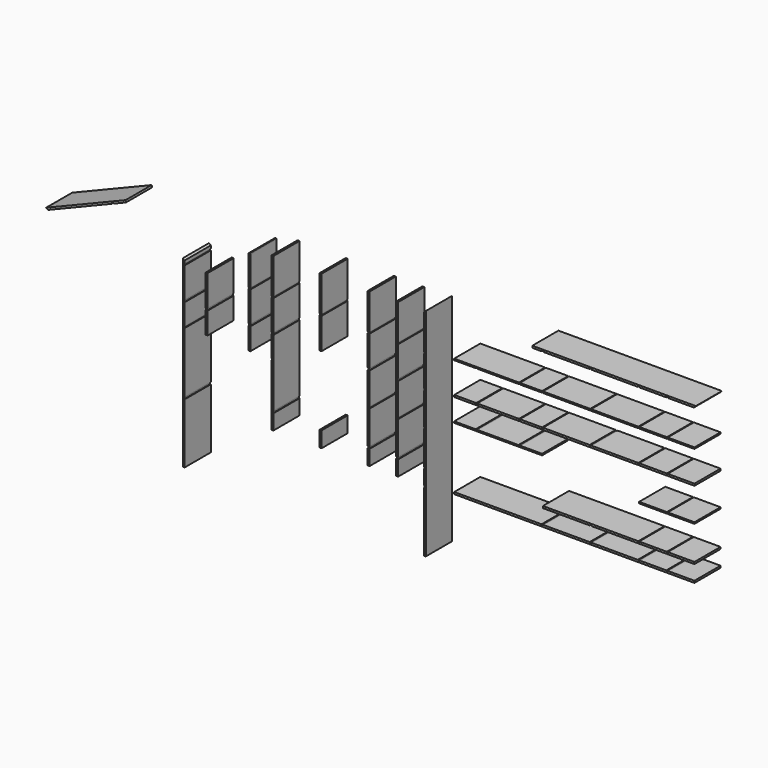
from build123d import *

# Parameters (mm, degrees)
F1_DEPTH = 400
F4_DEPTH = 400
F5_DEPTH = 400


# Not quite as in the source:
# - a feature names something its author has since deleted; it is built from what else it names


with BuildPart() as f1:
    # F0 (on Front) → F1 (new body)
    with BuildSketch(Plane.XZ):
        Polygon((0, 2251), (0, 0), (24, 0), (24, 502), (24, 735), (17, 735), (17, 759), (24, 759), (24, 1504.2), (17, 1504.2), (17, 1522.2), (24, 1522.2), (24, 1783), (17, 1783), (17, 1807), (24, 1807), (24, 2181), (17, 2181), (17, 2199), (24, 2199), (24, 2234.8896542695), align=None)
    extrude(amount=F1_DEPTH)


with BuildPart() as f1b:
    # F0 (on Front) → F1, piece 2 (new body)
    with BuildSketch(Plane.XZ):
        Polygon((2980, 0), (2980, 2650), (2956, 2626), (2956, 2249), (2956, 2199), (2963, 2199), (2963, 2181), (2956, 2181), (2956, 1807), (2963, 1807), (2963, 1783), (2956, 1783), (2956, 1390.5), (2963, 1390.5), (2963, 1372.5), (2956, 1372.5), (2956, 962), (2963, 962), (2963, 938), (2956, 938), (2956, 759), (2963, 759), (2963, 735), (2956, 735), (2956, 550), (2956, 526), (2956, 502), (2956, 0), align=None)
    extrude(amount=F1_DEPTH)


with BuildPart() as f1c:
    # F0 (on Front) → F1, piece 3 (new body)
    with BuildSketch(Plane.XZ):
        Polygon((804.639455329, 2565.1562908123), (804.639455329, 2554.3513390656), (804.6394553291, 2249), (804.6394553291, 2199), (811.639455329, 2199), (811.639455329, 2181), (804.6394553291, 2181), (804.6394553293, 1807), (811.639455329, 1807), (811.639455329, 1783), (804.6394553293, 1783), (804.6394553294, 1522.2), (804.6394553294, 1515.2), (828.6394553284, 1515.2), (828.6394553284, 1522.2), (828.6394553285, 1783), (821.6394553285, 1783), (821.6394553285, 1807), (828.6394553285, 1807), (828.6394553288, 2181), (821.6394553288, 2181), (821.6394553288, 2199), (828.6394553288, 2199), (828.6394553288, 2249), (828.639455329, 2564.1728775272), (824.8520180611, 2573.4278934073), align=None)
    extrude(amount=F1_DEPTH)


with BuildPart() as f1d:
    # F0 (on Front) → F1, piece 4 (new body)
    with BuildSketch(Plane.XZ):
        Polygon((1088, 2636), (1088, 2626), (1088, 2249), (1088, 2199), (1095, 2199), (1095, 2181), (1088, 2181), (1088, 1807), (1095, 1807), (1095, 1783), (1088, 1783), (1088, 1522.1999999999), (1095, 1522.1999999998), (1095, 1504.2), (1088, 1504.2), (1088, 1222.6), (1088, 938), (1088, 759), (1088, 752), (1112, 752), (1112, 759), (1112, 938), (1105, 938), (1105, 962), (1112, 962), (1112, 1222.6), (1112, 1783), (1105, 1783), (1105, 1807), (1112, 1807), (1112, 2181), (1105, 2181), (1105, 2199), (1112, 2199), (1112, 2249), (1112, 2626), (1112, 2636), align=None)
    extrude(amount=F1_DEPTH)


with BuildPart() as f1e:
    # F0 (on Front) → F1, piece 5 (new body)
    with BuildSketch(Plane.XZ):
        Polygon((2642, 2249), (2642, 2626), (2642, 2636), (2618, 2636), (2618, 2626), (2618, 2249), (2618, 2199), (2625, 2199), (2625, 2181), (2618, 2181), (2618, 1807), (2625, 1807), (2625, 1783), (2618, 1783), (2618, 1390.5), (2625, 1390.5), (2625, 1372.5), (2618, 1372.5), (2618, 962), (2625, 962), (2625, 938), (2618, 938), (2618, 759), (2618, 752), (2642, 752), (2642, 759), (2642, 938), (2635, 938), (2635, 962), (2642, 962), (2642, 1372.5), (2635, 1372.5), (2635, 1390.5), (2642, 1390.5), (2642, 1783), (2635, 1783), (2635, 1807), (2642, 1807), (2642, 2181), (2635, 2181), (2635, 2199), (2642, 2199), align=None)
    extrude(amount=F1_DEPTH)


with BuildPart() as f1f:
    # F0 (on Front) → F1, piece 6 (new body)
    with BuildSketch(Plane.XZ):
        Polygon((280.5054049087, 2188), (280.5054049087, 2181), (280.5054049087, 1807), (287.5054049087, 1807), (287.5054049087, 1783), (280.5054049087, 1783), (280.5054049087, 1522.2), (280.5054049087, 1515.2), (304.5054049087, 1515.2), (304.5054049087, 1522.2), (304.5054049087, 1783), (297.5054049087, 1783), (297.5054049087, 1807), (304.5054049087, 1807), (304.5054049087, 2181), (304.5054049087, 2188), align=None)
    extrude(amount=F1_DEPTH)


with BuildPart() as f1g:
    # F0 (on Front) → F1, piece 7 (new body)
    with BuildSketch(Plane.XZ):
        Polygon((1678, 2636), (1678, 2626), (1678, 2249), (1678, 2199), (1685, 2199), (1685, 2181), (1678, 2181), (1678, 1807), (1678, 1800), (1702, 1800), (1702, 1807), (1702, 2181), (1695, 2181), (1695, 2199), (1702, 2199), (1702, 2249), (1702, 2626), (1702, 2636), align=None)
    extrude(amount=F1_DEPTH)


with BuildPart() as f1h:
    # F0 (on Front) → F1, piece 8 (new body)
    with BuildSketch(Plane.XZ):
        Polygon((2291.9720954895, 2249), (2291.9720954895, 2626), (2291.9720954895, 2636), (2268, 2636), (2268, 2626), (2268, 2249), (2268, 2199), (2275, 2199), (2275, 2181), (2268, 2181), (2268, 1807), (2275, 1807), (2275, 1783), (2268, 1783), (2268, 962), (2275, 962), (2275, 938), (2268, 938), (2268, 759), (2268, 752), (2292, 752), (2292, 759), (2292, 938), (2284.9720954895, 938), (2284.9720954895, 962), (2292, 962), (2292, 1372.5), (2284.9720954895, 1372.5), (2284.9720954895, 1390.5), (2292, 1390.5), (2292, 1783), (2284.9720954895, 1783), (2284.9720954895, 1807), (2291.9720954895, 1807), (2291.9720954895, 2181), (2284.9720954895, 2181), (2284.9720954895, 2199), (2291.9720954895, 2199), align=None)
    extrude(amount=F1_DEPTH)


with BuildPart() as f1i:
    # F0 (on Front) → F1, piece 9 (new body)
    with BuildSketch(Plane.XZ):
        Polygon((1678, 938), (1678, 759), (1678, 752), (1702, 752), (1702, 759), (1702, 938), (1702, 945), (1678, 945), align=None)
    extrude(amount=F1_DEPTH)


with BuildPart() as f4:
    # F3 (on Front) → F4 (new body)
    with BuildSketch(Plane.XZ):
        Polygon((-701.0374307632, 2650), (-1676.0374307632, 2251), (-1652.0374307632, 2234.8896542695), (-871.3979754343, 2554.3513390656), (-871.3979754343, 2565.1562908123), (-851.1854127022, 2573.4278934073), (-847.3979754343, 2564.1728775272), (-696.3166611209, 2626), align=None)
    extrude(amount=F4_DEPTH)


with BuildPart() as f5:
    # F2 (on Front) → F5 (new body)
    with BuildSketch(Plane.XZ):
        Polygon((6291.6567134857, 2700.713174873), (4286.6567134857, 2700.713174873), (4289.0170983069, 2688.713174873), (4291.377483128, 2676.713174873), (4399.6567134857, 2676.713174873), (4399.6567134857, 2686.713174873), (4423.6567134857, 2686.713174873), (4423.6567134857, 2676.713174873), (4989.6567134857, 2676.713174873), (4989.6567134857, 2686.713174873), (5013.6567134857, 2686.713174873), (5013.6567134857, 2676.713174873), (5579.6567134857, 2676.713174873), (5579.6567134857, 2686.713174873), (5603.6288089752, 2686.713174873), (5603.6288089752, 2676.713174873), (5929.6567134857, 2676.713174873), (5929.6567134857, 2686.713174873), (5953.6567134857, 2686.713174873), (5953.6567134857, 2676.713174873), (6267.6567134857, 2676.713174873), align=None)
    extrude(amount=F5_DEPTH)


with BuildPart() as f5b:
    # F2 (on Front) → F5, piece 2 (new body)
    with BuildSketch(Plane.XZ):
        Polygon((5953.6567134857, 988.713174873), (6267.6567134857, 988.713174873), (6274.6567134857, 988.713174873), (6274.6567134857, 1012.713174873), (6267.6567134857, 1012.713174873), (6129.7695007324, 1012.713174873), (5953.6567134857, 1012.713174873), (5946.6567134857, 1012.713174873), (5946.6567134857, 988.713174873), align=None)
    extrude(amount=F5_DEPTH)


with BuildPart() as f5c:
    # F2 (on Front) → F5, piece 3 (new body)
    with BuildSketch(Plane.XZ):
        Polygon((5603.6567134857, 988.713174873), (5929.6567134857, 988.713174873), (5936.6567134857, 988.713174873), (5936.6567134857, 1012.713174873), (5929.6567134857, 1012.713174873), (5603.6567134857, 1012.713174873), (5596.6288089752, 1012.713174873), (5596.6288089752, 988.713174873), align=None)
    extrude(amount=F5_DEPTH)


with BuildPart() as f5d:
    # F2 (on Front) → F5, piece 4 (new body)
    with BuildSketch(Plane.XZ):
        Polygon((4416.6567134857, 988.713174873), (4423.6567134857, 988.713174873), (4989.6567134857, 988.713174873), (4989.6567134857, 995.713174873), (5013.6567134857, 995.713174873), (5013.6567134857, 988.713174873), (5579.6567134857, 988.713174873), (5586.6567134857, 988.713174873), (5586.6567134857, 1012.713174873), (5579.6567134857, 1012.713174873), (4423.6567134857, 1012.713174873), (4416.6567134857, 1012.713174873), align=None)
    extrude(amount=F5_DEPTH)


with BuildPart() as f5e:
    # F2 (on Front) → F5, piece 5 (new body)
    with BuildSketch(Plane.XZ):
        Polygon((5603.6567134857, 1423.213174873), (5929.6567134857, 1423.213174873), (5936.6567134857, 1423.213174873), (5936.6567134857, 1441.213174873), (5929.6567134857, 1441.213174873), (5603.6567134857, 1441.213174873), (5596.6288089752, 1441.213174873), (5596.6288089752, 1423.213174873), align=None)
    extrude(amount=F5_DEPTH)


with BuildPart() as f5f:
    # F2 (on Front) → F5, piece 6 (new body)
    with BuildSketch(Plane.XZ):
        Polygon((5953.6567134857, 1423.213174873), (6267.6567134857, 1423.213174873), (6274.6567134857, 1423.213174873), (6274.6567134857, 1441.213174873), (6267.6567134857, 1441.213174873), (5953.6567134857, 1441.213174873), (5946.6567134857, 1441.213174873), (5946.6567134857, 1423.213174873), align=None)
    extrude(amount=F5_DEPTH)


with BuildPart() as f5g:
    # F2 (on Front) → F5, piece 7 (new body)
    with BuildSketch(Plane.XZ):
        Polygon((6274.6567134857, 1857.713174873), (6267.6567134857, 1857.713174873), (5953.6567134857, 1857.713174873), (5946.6567134857, 1857.713174873), (5946.6567134857, 1833.713174873), (5953.6567134857, 1833.713174873), (6129.7695007324, 1833.713174873), (6267.6567134857, 1833.713174873), (6274.6567134857, 1833.713174873), align=None)
    extrude(amount=F5_DEPTH)


with BuildPart() as f5h:
    # F2 (on Front) → F5, piece 8 (new body)
    with BuildSketch(Plane.XZ):
        Polygon((5936.6567134857, 1857.713174873), (5929.6567134857, 1857.713174873), (5603.6288089752, 1857.713174873), (5596.6288089752, 1857.713174873), (5596.6288089752, 1833.713174873), (5603.6567134857, 1833.713174873), (5929.6567134857, 1833.713174873), (5936.6567134857, 1833.713174873), align=None)
    extrude(amount=F5_DEPTH)


with BuildPart() as f5i:
    # F2 (on Front) → F5, piece 9 (new body)
    with BuildSketch(Plane.XZ):
        Polygon((4989.6567134857, 1857.713174873), (4423.6567134857, 1857.713174873), (4416.6567134857, 1857.713174873), (4416.6567134857, 1833.713174873), (4423.6567134857, 1833.713174873), (5579.6567134857, 1833.713174873), (5586.6567134857, 1833.713174873), (5586.6567134857, 1857.713174873), (5579.6567134857, 1857.713174873), (5013.6567134857, 1857.713174873), (5013.6567134857, 1850.713174873), (4989.6567134857, 1850.713174873), align=None)
    extrude(amount=F5_DEPTH)


with BuildPart() as f5j:
    # F2 (on Front) → F5, piece 10 (new body)
    with BuildSketch(Plane.XZ):
        Polygon((3328.6567134857, 1554.913174873), (3335.6567134857, 1554.913174873), (4399.6567134857, 1554.913174873), (4406.6567134857, 1554.913174873), (4406.6567134857, 1572.913174873), (4399.6567134857, 1572.913174873), (4140.2961688146, 1572.913174873), (4140.2961688146, 1565.913174873), (4116.2961688147, 1565.913174873), (4116.2961688147, 1572.913174873), (3616.1621183944, 1572.913174873), (3616.1621183944, 1565.913174873), (3592.1621183944, 1565.913174873), (3592.1621183944, 1572.913174873), (3335.6567134857, 1572.913174873), (3328.6567134857, 1572.913174873), align=None)
    extrude(amount=F5_DEPTH)


with BuildPart() as f5k:
    # F2 (on Front) → F5, piece 11 (new body)
    with BuildSketch(Plane.XZ):
        Polygon((4123.2961688147, 1857.713174873), (4116.2961688147, 1857.713174873), (3616.1621183944, 1857.713174873), (3610.326230526, 1857.713174873), (3610.326230526, 1833.713174873), (3616.1621183944, 1833.713174873), (4116.2961688147, 1833.713174873), (4123.2961688147, 1833.713174873), align=None)
    extrude(amount=F5_DEPTH)


with BuildPart() as f5l:
    # F2 (on Front) → F5, piece 12 (new body)
    with BuildSketch(Plane.XZ):
        Polygon((3592.1621183944, 1857.713174873), (3335.6567134857, 1857.713174873), (3328.6567134857, 1857.713174873), (3328.6567134857, 1833.713174873), (3335.6567134857, 1833.713174873), (3592.1621183944, 1833.713174873), (3598.9656448364, 1833.713174873), (3598.9656448364, 1857.713174873), align=None)
    extrude(amount=F5_DEPTH)


with BuildPart() as f5m:
    # F2 (on Front) → F5, piece 13 (new body)
    with BuildSketch(Plane.XZ):
        Polygon((3610.326230526, 2249.7131748731), (3335.6567134857, 2249.7131748731), (3328.6567134857, 2249.7131748731), (3328.6567134857, 2231.713174873), (3335.6567134857, 2231.713174873), (3592.1621183945, 2231.713174873), (3592.1621183945, 2238.713174873), (3616.1621183945, 2238.713174873), (3616.1621183945, 2231.713174873), (4116.2961688147, 2231.713174873), (4123.2961688147, 2231.713174873), (4123.2961688147, 2249.7131748731), (4116.2961688147, 2249.7131748731), align=None)
    extrude(amount=F5_DEPTH)


with BuildPart() as f5n:
    # F2 (on Front) → F5, piece 14 (new body)
    with BuildSketch(Plane.XZ):
        Polygon((4989.6567134857, 2249.7131748731), (4423.6567134857, 2249.7131748731), (4416.6567134857, 2249.7131748731), (4416.6567134857, 2231.713174873), (4423.6567134857, 2231.713174873), (4989.6567134857, 2231.713174873), (4996.6567134857, 2231.713174873), (4996.6567134857, 2249.7131748731), align=None)
    extrude(amount=F5_DEPTH)


with BuildPart() as f5o:
    # F2 (on Front) → F5, piece 15 (new body)
    with BuildSketch(Plane.XZ):
        Polygon((5586.6567134857, 2249.7131748731), (5579.6567134857, 2249.7131748731), (5013.6567134857, 2249.7131748731), (5006.6567134857, 2249.7131748731), (5006.6567134857, 2231.713174873), (5013.6567134857, 2231.713174873), (5579.6567134857, 2231.713174873), (5586.6567134857, 2231.713174873), align=None)
    extrude(amount=F5_DEPTH)


with BuildPart() as f5p:
    # F2 (on Front) → F5, piece 16 (new body)
    with BuildSketch(Plane.XZ):
        Polygon((5936.6567134857, 2249.713174873), (5929.6567134857, 2249.713174873), (5603.6288089752, 2249.7131748731), (5596.6288089752, 2249.7131748731), (5596.6288089752, 2231.713174873), (5603.6288089752, 2231.713174873), (5929.6567134857, 2231.7131748729), (5936.6567134857, 2231.7131748729), align=None)
    extrude(amount=F5_DEPTH)


with BuildPart() as f5q:
    # F2 (on Front) → F5, piece 17 (new body)
    with BuildSketch(Plane.XZ):
        Polygon((6274.6567134857, 2249.713174873), (6267.6567134857, 2249.713174873), (5953.6567134857, 2249.713174873), (5946.6567134857, 2249.713174873), (5946.6567134857, 2231.7131748729), (5953.6567134857, 2231.7131748729), (6267.6567134857, 2231.7131748729), (6274.6567134857, 2231.7131748729), align=None)
    extrude(amount=F5_DEPTH)


with BuildPart() as f5r:
    # F2 (on Front) → F5, piece 18 (new body)
    with BuildSketch(Plane.XZ):
        Polygon((3328.6567134857, 785.713174873), (3335.6567134857, 785.713174873), (6267.6567134857, 785.713174873), (6274.6567134857, 785.713174873), (6274.6567134857, 809.713174873), (6267.6567134857, 809.713174873), (5953.6567134857, 809.713174873), (5953.6567134857, 802.713174873), (5929.6567134857, 802.713174873), (5929.6567134857, 809.713174873), (5603.6567134857, 809.713174873), (5603.6567134857, 802.713174873), (5579.6567134857, 802.713174873), (5579.6567134857, 809.713174873), (5013.6567134857, 809.713174873), (5013.6567134857, 802.713174873), (4989.6567134857, 802.713174873), (4989.6567134857, 809.713174873), (4423.6567134857, 809.713174873), (4423.6567134857, 802.713174873), (4399.6567134857, 802.713174873), (4399.6567134857, 809.713174873), (3335.6567134857, 809.713174873), (3328.6567134857, 809.713174873), align=None)
    extrude(amount=F5_DEPTH)


with BuildPart() as f5s:
    # F2 (on Front) → F5, piece 19 (new body)
    with BuildSketch(Plane.XZ):
        Polygon((4406.6567134857, 2249.7131748731), (4399.6567134857, 2249.7131748731), (4140.2961688147, 2249.7131748731), (4133.2947083473, 2249.7131748731), (4133.2947083473, 2231.713174873), (4140.2961688147, 2231.713174873), (4399.6567134857, 2231.713174873), (4406.6567134857, 2231.713174873), align=None)
    extrude(amount=F5_DEPTH)


with BuildPart() as f5t:
    # F2 (on Front) → F5, piece 20 (new body)
    with BuildSketch(Plane.XZ):
        Polygon((4406.6567134857, 1857.713174873), (4399.6567134857, 1857.713174873), (4140.2961688146, 1857.713174873), (4133.2947083473, 1857.713174873), (4133.2947083473, 1833.713174873), (4140.2961688146, 1833.713174873), (4399.6567134857, 1833.713174873), (4406.6567134857, 1833.713174873), align=None)
    extrude(amount=F5_DEPTH)


solid = Compound([f1.part, f1b.part, f1c.part, f1d.part, f1e.part, f1f.part, f1g.part, f1h.part, f1i.part, f4.part, f5.part, f5b.part, f5c.part, f5d.part, f5e.part, f5f.part, f5g.part, f5h.part, f5i.part, f5j.part, f5k.part, f5l.part, f5m.part, f5n.part, f5o.part, f5p.part, f5q.part, f5r.part, f5s.part, f5t.part])
